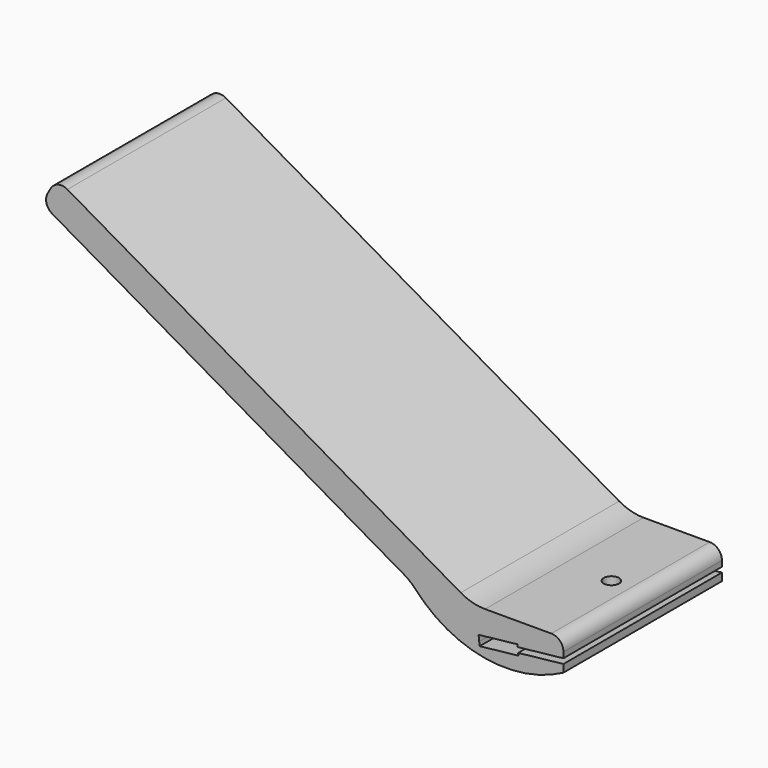
from build123d import *

# Parameters (mm, degrees)
F1_DEPTH = 41.275
F2_R     = 1.6
F2_R_2   = 1.25
F3_DEPTH = 4.6024929371
F4_DEPTH = 9.3840608367
F6_R     = 10.16
F7_R     = 2.54


with BuildPart() as f1:
    # F0 (on Front) → F1 (new body)
    with BuildSketch(Plane.XZ):
        Polygon((-10.9985226281, 6.35), (0, 0), (3.1994554543, 0), (3.0682228412, 1.200819531), (11.1481153525, 2.0838376541), (11.2019242694, 1.5914692042), (20.7514773719, 2.6351004709), (20.7514773719, 6.35), (1.7014773719, 6.35), (-84.8131810245, 56.299261314), (-87.9881810245, 50.8), align=None)
        with BuildLine():
            Line((3.1994554543, 0), (0, 0))
            Line((0, 0), (-10.9985226281, 6.35))
            ThreePointArc((-10.9985226281, 6.35), (3.7335153721, -2.5398099993), (20.7514773719, 0))
            Line((20.7514773719, 0), (10.7844894565, 0))
            Line((10.7844894565, 0), (3.2889773719, -0.8191535968))
            Line((3.2889773719, -0.8191535968), (3.1994554543, 0))
        make_face()
        Polygon((10.7844894565, 0), (20.7514773719, 0), (20.7514773719, 1.5875), (11.3150609664, 0.5562329762), (11.3688698832, 0.0638645263), align=None)
    extrude(amount=F1_DEPTH)

    # F2 (on face) → F3 (cut, through all)
    with BuildSketch(Plane.XY.offset(6.35)):
        with Locations((14.2388698832, -20.6375)):
            Circle(F2_R)
        with Locations((14.2388698832, -20.6375)):
            Circle(F2_R_2, mode=Mode.SUBTRACT)
        with Locations((14.2388698832, -20.6375)):
            Circle(F2_R_2)
    extrude(amount=-F3_DEPTH, mode=Mode.SUBTRACT)

    # F2 (on face) → F4 (cut, through all)
    with BuildSketch(Plane.XY.offset(6.35)):
        with Locations((14.2388698832, -20.6375)):
            Circle(F2_R_2)
    extrude(amount=-F4_DEPTH, mode=Mode.SUBTRACT)

    # F6
    f6_edges = [f1.edges().sort_by_distance(p)[0] for p in [
        (-10.998523, -20.6375, 6.35),
        (1.701477, -20.6375, 6.35),
    ]]
    fillet(f6_edges, radius=F6_R)

    # F7
    f7_edges = [f1.edges().sort_by_distance(p)[0] for p in [
        (-87.988181, -20.6375, 50.8),
        (-84.813181, -20.6375, 56.299261),
        (20.751477, -20.6375, 6.35),
    ]]
    fillet(f7_edges, radius=F7_R)


solid = f1.part
